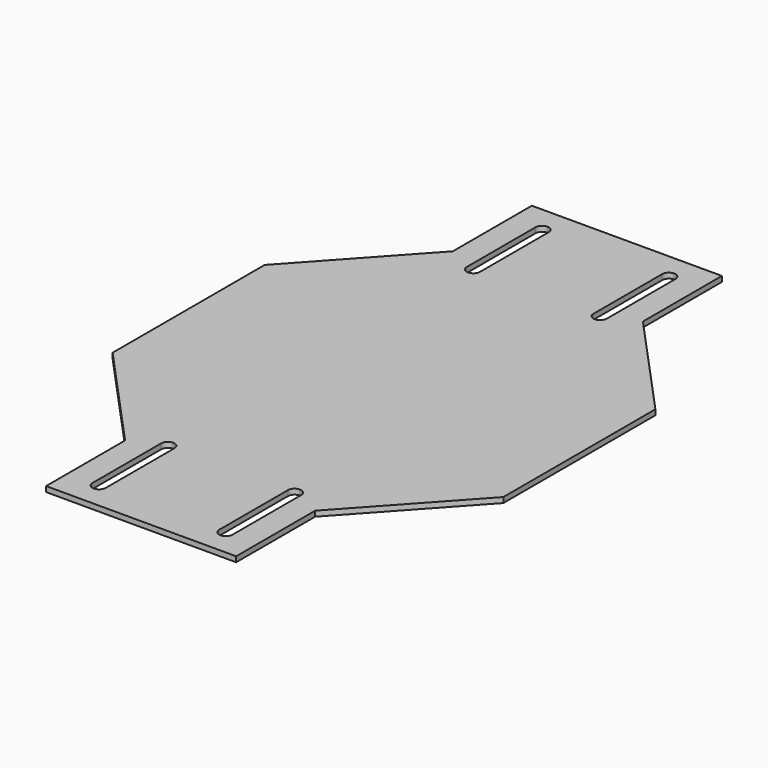
from build123d import *

# Parameters (mm, degrees)
F0_W     = 30.1625
F0_H     = 57.15
F0_W_2   = 57.15
F1_DEPTH = 1.6002
F3_DEPTH = 1.6012


with BuildPart() as f1:
    # F0 (on Top) → F1 (new body)
    with BuildSketch(Plane.XY):
        Polygon((57.15, 62.70625), (57.15, 29.68625), (87.3125, 62.70625), align=None)
        Polygon((-30.1625, 62.70625), (0, 29.68625), (0, 62.70625), align=None)
        Polygon((57.15, 152.87625), (57.15, 119.85625), (87.3125, 119.85625), align=None)
        Polygon((-30.1625, 119.85625), (0, 119.85625), (0, 152.87625), align=None)
        Polygon((0, 29.68625), (0, 0), (57.15, 0), (57.15, 29.68625), (57.15, 62.70625), (0, 62.70625), align=None)
        with Locations((-15.08125, 91.28125)):
            Rectangle(F0_W, F0_H)
        with Locations((72.23125, 91.28125)):
            Rectangle(F0_W, F0_H)
        with Locations((28.575, 91.28125)):
            Rectangle(F0_W_2, F0_H)
        Polygon((0, 152.87625), (0, 119.85625), (57.15, 119.85625), (57.15, 152.87625), (57.15, 182.5625), (0, 182.5625), align=None)
    extrude(amount=F1_DEPTH)

    # F2 (on face) → F3 (cut, through all)
    with BuildSketch(Plane.XY.offset(1.6002)):
        with BuildLine():
            ThreePointArc((11.52525, 174.52975), (10.9393903391, 175.9441403391), (9.525, 176.53))
            ThreePointArc((9.525, 176.53), (8.1106096609, 175.9441403391), (7.52475, 174.52975))
            Line((7.52475, 174.52975), (7.52475, 148.71065))
            ThreePointArc((7.52475, 148.71065), (8.1106096609, 147.2962596609), (9.525, 146.7104))
            ThreePointArc((9.525, 146.7104), (10.9393903391, 147.2962596609), (11.52525, 148.71065))
            Line((11.52525, 148.71065), (11.52525, 174.52975))
        make_face()
        with BuildLine():
            ThreePointArc((49.62525, 174.52975), (49.0393903391, 175.9441403391), (47.625, 176.53))
            ThreePointArc((47.625, 176.53), (46.2106096609, 175.9441403391), (45.62475, 174.52975))
            Line((45.62475, 174.52975), (45.62475, 148.71065))
            ThreePointArc((45.62475, 148.71065), (46.2106096609, 147.2962596609), (47.625, 146.7104))
            ThreePointArc((47.625, 146.7104), (49.0393903391, 147.2962596609), (49.62525, 148.71065))
            Line((49.62525, 148.71065), (49.62525, 174.52975))
        make_face()
        with BuildLine():
            ThreePointArc((7.52475, 8.03275), (8.1106096609, 6.6183596609), (9.525, 6.0325))
            ThreePointArc((9.525, 6.0325), (10.9393903391, 6.6183596609), (11.52525, 8.03275))
            Line((11.52525, 8.03275), (11.52525, 33.85185))
            ThreePointArc((11.52525, 33.85185), (10.9393903391, 35.2662403391), (9.525, 35.8521))
            ThreePointArc((9.525, 35.8521), (8.1106096609, 35.2662403391), (7.52475, 33.85185))
            Line((7.52475, 33.85185), (7.52475, 8.03275))
        make_face()
        with BuildLine():
            ThreePointArc((45.62475, 8.03275), (46.2106096609, 6.6183596609), (47.625, 6.0325))
            ThreePointArc((47.625, 6.0325), (49.0393903391, 6.6183596609), (49.62525, 8.03275))
            Line((49.62525, 8.03275), (49.62525, 33.85185))
            ThreePointArc((49.62525, 33.85185), (49.0393903391, 35.2662403391), (47.625, 35.8521))
            ThreePointArc((47.625, 35.8521), (46.2106096609, 35.2662403391), (45.62475, 33.85185))
            Line((45.62475, 33.85185), (45.62475, 8.03275))
        make_face()
    extrude(amount=-F3_DEPTH, mode=Mode.SUBTRACT)


solid = f1.part
